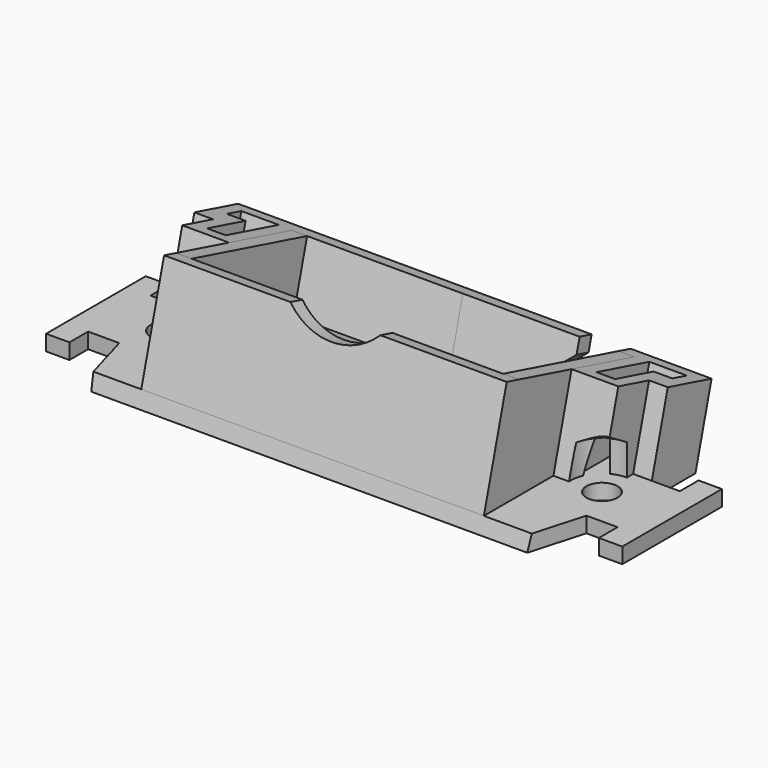
from build123d import *

# Parameters (mm, degrees)
F1_DEPTH  = 1
F3_DEPTH  = 11
F4_DEPTH  = 10
F5_W      = 1.2
F5_H      = 0.6395594371
F6_REACH  = 15.595486632
F7_SIZE2  = 0.267939
F7_SIZE   = 0.99999
F8_D      = 2
F8_DEPTH  = 2
F8_TIP    = 0.600860619
F10_D     = 5
F10_DEPTH = 5
F10_TIP   = 1.5021515476
F11_D     = 4
F11_DEPTH = 2
F11_TIP   = 1.2017212381
F14_DEPTH = 1
F16_DEPTH = 1


# Not quite as in the source:
# - a fillet or chamfer is up to 0.001 mm smaller than in the source, because OpenCascade refuses the exact size
# - a feature names something its author has since deleted; it is built from what else it names


with BuildPart() as f1:
    # F0 (on Top) → F1 (new body)
    with BuildSketch(Plane.XY):
        Polygon((-18.5, 4), (-18.5, 0), (-18.5, -4), (-17, -4), (-17, -2.5), (-15, -2.5), (-14, -6), (0, -6), (0, 6), (-10.2, 6), (-10.2, -0.1), (-13.1, -0.1), (-13.1, 3.1), (-14.4, 3.1), (-14.4, 6), (-15, 2.5), (-17, 2.5), (-17, 4), align=None)
        Polygon((-10.2, 6), (-14.4, 6), (-14.4, 3.1), (-13.1, 3.1), (-13.1, -0.1), (-10.2, -0.1), align=None)
        Polygon((-11, 5.2), (-11, 0.7), (-12.3, 0.7), (-12.3, 3.9), (-13.6, 3.9), (-13.6, 5.2), align=None, mode=Mode.SUBTRACT)
        Polygon((-12.3, 0.7), (-11, 0.7), (-11, 5.2), (-13.6, 5.2), (-13.6, 3.9), (-12.3, 3.9), align=None)
    extrude(amount=F1_DEPTH)

    # F2 (on Right) → F3 (join)
    with BuildSketch(Plane.YZ):
        Polygon((-6, 0), (-4.9647238196, 0), (-4.0316277581, 3.4823619098), (-2.9361313709, 7.5708100863), (-3.9020571972, 7.8296291314), align=None)
        Polygon((4.9647238196, 0), (6, 0), (7.2940952255, 4.8296291314), (6.3281693992, 5.0884481765), (5.232673012, 1), align=None)
        Polygon((-4.9647238196, 0), (4.9647238196, 0), (5.232673012, 1), (-4.0316277581, 3.4823619098), align=None)
        Polygon((-4.0316277581, 3.4823619098), (5.232673012, 1), (6.3281693992, 5.0884481765), (-2.9361313709, 7.5708100863), align=None)
    extrude(amount=-F3_DEPTH)

    # F2 (on Right) → F4 (cut)
    with BuildSketch(Plane.YZ):
        Polygon((-4.0316277581, 3.4823619098), (5.232673012, 1), (6.3281693992, 5.0884481765), (-2.9361313709, 7.5708100863), align=None)
    extrude(amount=-F4_DEPTH, mode=Mode.SUBTRACT)

    f6_end = Plane(origin=(-8.4427376171, 0.0169846051, 0), x_dir=(-1, 0, 0), z_dir=(0, 0, -1))
    # F5 (on face) → F6 (join, up to a plane its end follows)
    with BuildSketch(Plane(origin=(0, 1.6960190142, 6.3296291314), x_dir=(1, 0, 0), z_dir=(0, 0.2588190451, 0.9659258263))):
        Polygon((-15.2, 5.7955549577), (-15.2, 2.7955549577), (-14, 2.7955549577), (-14, 2.1559955206), (-14, -0.4044450423), (-11, -0.4044450423), (-11, 5.7955549577), align=None)
        Polygon((-11.9, 4.8955549577), (-11.9, 0.4955549577), (-13.1, 0.4955549577), (-13.1, 3.6955549577), (-14.3, 3.6955549577), (-14.3, 4.8955549577), align=None, mode=Mode.SUBTRACT)
        with Locations((-14.6, 2.4757752392)):
            Rectangle(F5_W, F5_H)
    f6_long = extrude(amount=-F6_REACH, mode=Mode.PRIVATE)
    add(split(f6_long, bisect_by=f6_end, keep=Keep.BOTTOM, mode=Mode.PRIVATE))

    # F7 (size 1 and 0.2679491924 in the source; OpenCascade refuses exactly that, so slightly less here)
    f7_edges = [f1.edges().sort_by_distance(p)[0] for p in [
        (-7, -6, 1),
    ]]
    f7_side = f1.faces().sort_by_distance((-7, -6, 0.5))[0]
    chamfer(f7_edges, length=F7_SIZE, length2=F7_SIZE2, reference=f7_side)

    # F8
    with Locations(Plane(origin=(0, 0, 0), x_dir=(1, 0, 0), z_dir=(0, 0, -1))):
        with Locations((-14, 0)):
            Hole(F8_D / 2, depth=F8_DEPTH)
            with Locations((0, 0, -(F8_DEPTH + F8_TIP / 2))):  # 118° drill point
                Cone(0, F8_D / 2, F8_TIP, mode=Mode.SUBTRACT)

    # F10
    with Locations(Plane(origin=(0, 0, 0), x_dir=(1, 0, 0), z_dir=(0, 0, -1))):
        with Locations((-6.7131645046, 0), (0, 0)):
            Hole(F10_D / 2, depth=F10_DEPTH)
            with Locations((0, 0, -(F10_DEPTH + F10_TIP / 2))):  # 118° drill point
                Cone(0, F10_D / 2, F10_TIP, mode=Mode.SUBTRACT)

    # F11 (one way)
    with BuildSketch(Plane(origin=(0, 0, 1), x_dir=(1, 0, 0), z_dir=(0, 0, -1))):
        with Locations((-14, 0)):
            Circle(F11_D / 2)
    extrude(amount=-F11_DEPTH, mode=Mode.SUBTRACT)
    with Locations(Plane(origin=(0, 0, 1), x_dir=(1, 0, 0), z_dir=(0, 0, -1))):
        with Locations((-14, 0)):
            with Locations((0, 0, -(F11_DEPTH + F11_TIP / 2))):  # 118° drill point
                Cone(0, F11_D / 2, F11_TIP, mode=Mode.SUBTRACT)

    # F12: F1 across plane


with BuildPart() as f1_1:
    add(f1.part)
    add(f1.part.mirror(Plane.YZ))

    # F13 (on face) → F14 (cut)
    with BuildSketch(Plane(origin=(0, -5.5980762114, 1.5), x_dir=(1, 0, 0), z_dir=(0, -0.9659258263, 0.2588190451))):
        with BuildLine():
            Line((0, 6.5529142706), (-2.8882349873, 6.5529142706))
            ThreePointArc((-2.8882349873, 6.5529142706), (0, 5.3202412586), (2.8882349873, 6.5529142706))
            Line((2.8882349873, 6.5529142706), (0, 6.5529142706))
        make_face()
    extrude(amount=-F14_DEPTH, mode=Mode.SUBTRACT)

    # F15 (on face) → F16 (cut, through all)
    with BuildSketch(Plane(origin=(0, 5.5980762114, -1.5), x_dir=(-1, 0, 0), z_dir=(0, 0.9659258263, -0.2588190451))):
        Polygon((-7.5, 6.5529142706), (-10, 6.5529142706), (-10, 2.3202412586), (-6, 2.3202412586), (-6, 4.3202412586), (-7.5, 5.5958246812), align=None)
    extrude(amount=-F16_DEPTH, mode=Mode.SUBTRACT)


solid = f1_1.part
